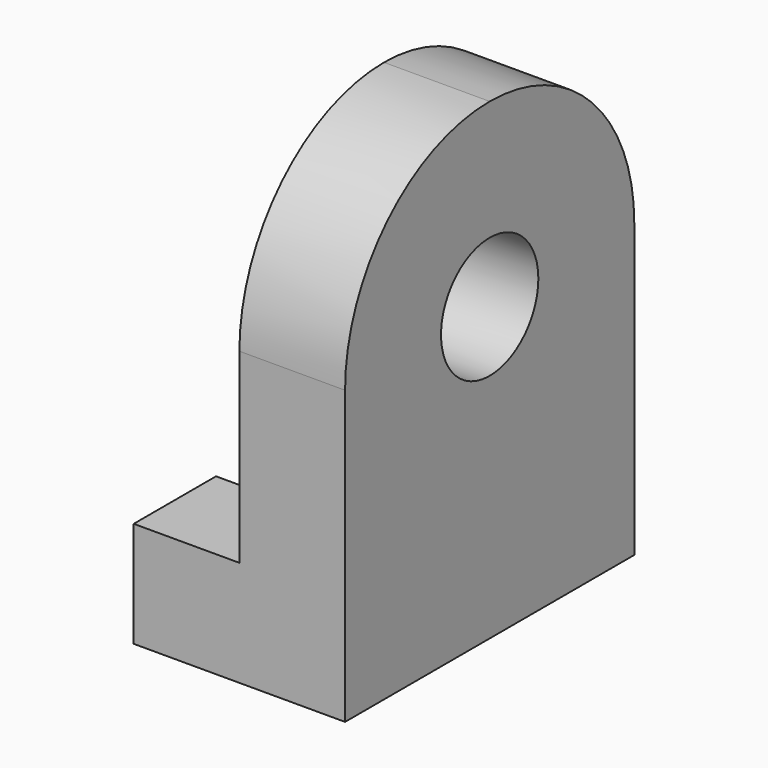
from build123d import *

# Parameters (mm, degrees)
F1_DEPTH = 66.04
F2_R     = 33.01999
F4_D     = 22.225
F4_DEPTH = 50.8
F4_TIP   = 6.6770636289
F5_W     = 9.652
F5_H     = 28.448
F6_DEPTH = 25.4


# Not quite as in the source:
# - a fillet or chamfer is up to 0.001 mm smaller than in the source, because OpenCascade refuses the exact size


with BuildPart() as f1:
    # F0 (on Front) → F1 (new body)
    with BuildSketch(Plane.XZ):
        Polygon((19.304, 0), (0, 0), (0, -19.304), (38.608, -19.304), (38.608, 67.056), (19.304, 67.056), align=None)
    extrude(amount=F1_DEPTH)

    # F2 (radius 33.02 in the source; OpenCascade refuses exactly that, so slightly less here)
    f2_edges = [f1.edges().sort_by_distance(p)[0] for p in [
        (28.956, 0, 67.056),
        (28.956, -66.04, 67.056),
    ]]
    fillet(f2_edges, radius=F2_R)

    # F4
    with Locations(Plane(origin=(19.304, 0, 0), x_dir=(0, -1, 0), z_dir=(-1, 0, 0))):
        with Locations((33.02, 34.036)):
            Hole(F4_D / 2, depth=F4_DEPTH)
            with Locations((0, 0, -(F4_DEPTH + F4_TIP / 2))):  # 118° drill point
                Cone(0, F4_D / 2, F4_TIP, mode=Mode.SUBTRACT)

    # F5 (on face) → F6 (cut)
    with BuildSketch(Plane.XY):
        with Locations((4.826, -33.02)):
            Rectangle(F5_W, F5_H)
    extrude(amount=-F6_DEPTH, mode=Mode.SUBTRACT)


solid = f1.part
